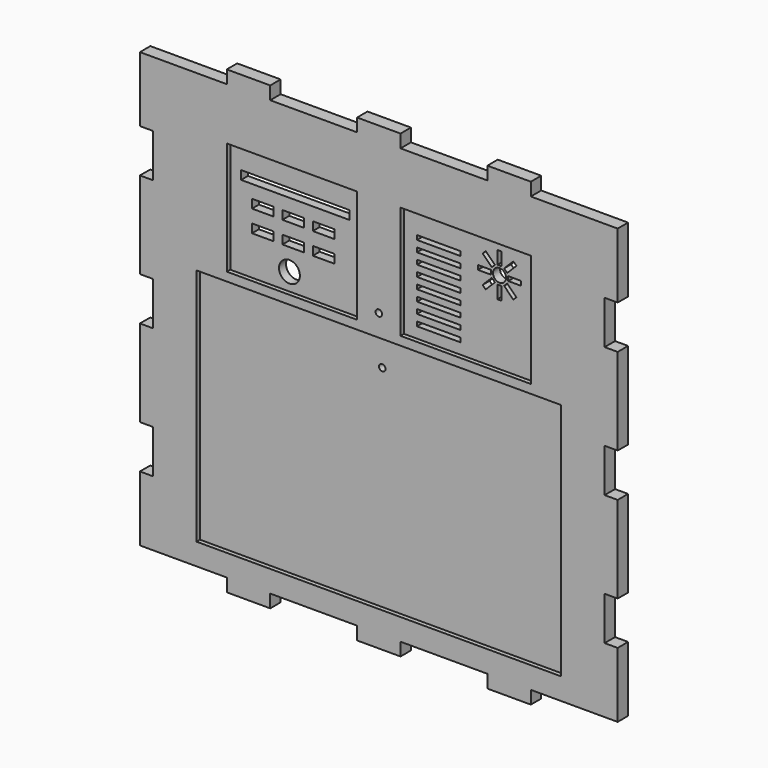
from build123d import *

# Parameters (mm, degrees)
F0_W     = 10
F0_H     = 3
F1_DEPTH = 3
F2_R     = 0.75
F2_W     = 5
F2_H     = 2
F2_R_2   = 2.4
F2_W_2   = 25
F2_W_3   = 10
F2_H_2   = 1
F2_R_3   = 1.5
F3_DEPTH = 3
F2_W_4   = 30
F2_H_3   = 26
F4_DEPTH = 1


# Not quite as in the source:
# - a feature names something its author has since deleted; it is built from what else it names


with BuildPart() as f1:
    # F0 (on Front) → F1 (new body)
    with BuildSketch(Plane.XZ):
        with Locations((-30, 51.5)):
            Rectangle(F0_W, F0_H)
        with Locations((0, 51.5)):
            Rectangle(F0_W, F0_H)
        with Locations((30, 51.5)):
            Rectangle(F0_W, F0_H)
        with Locations((-30, 48.5)):
            Rectangle(F0_W, F0_H)
        with Locations((0, 48.5)):
            Rectangle(F0_W, F0_H)
        with Locations((30, 48.5)):
            Rectangle(F0_W, F0_H)
        Polygon((-35, 50), (-55, 50), (-55, 35), (-52, 35), (-52, 25), (-55, 25), (-55, 5), (-52, 5), (-52, -5), (-55, -5), (-55, -25), (-52, -25), (-52, -35), (-55, -35), (-55, -50), (-35, -50), (-35, -47), (-25, -47), (-25, -50), (-5, -50), (-5, -47), (5, -47), (5, -50), (25, -50), (25, -47), (35, -47), (35, -50), (55, -50), (55, -35), (52, -35), (52, -25), (55, -25), (55, -5), (52, -5), (52, 5), (55, 5), (55, 25), (52, 25), (52, 35), (55, 35), (55, 50), (35, 50), (35, 47), (25, 47), (25, 50), (5, 50), (5, 47), (-5, 47), (-5, 50), (-25, 50), (-25, 47), (-35, 47), align=None)
        with Locations((30, -48.5)):
            Rectangle(F0_W, F0_H)
        with Locations((30, -51.5)):
            Rectangle(F0_W, F0_H)
        with Locations((0, -48.5)):
            Rectangle(F0_W, F0_H)
        with Locations((0, -51.5)):
            Rectangle(F0_W, F0_H)
        with Locations((-30, -48.5)):
            Rectangle(F0_W, F0_H)
        with Locations((-30, -51.5)):
            Rectangle(F0_W, F0_H)
    extrude(amount=F1_DEPTH)

    # F2 (on face) → F3 (cut)
    with BuildSketch(Plane.XZ.offset(3)):
        with Locations((0, 15)):
            Circle(F2_R)
        with Locations((-13.5, 22)):
            Rectangle(F2_W, F2_H)
        with Locations((-20.5, 22)):
            Rectangle(F2_W, F2_H)
        with Locations((-21.369388327, 16)):
            Circle(F2_R_2)
        with Locations((-27.5, 22)):
            Rectangle(F2_W, F2_H)
        with Locations((-27.5, 27)):
            Rectangle(F2_W, F2_H)
        with Locations((-20.5, 27)):
            Rectangle(F2_W, F2_H)
        with Locations((-13.5, 27)):
            Rectangle(F2_W, F2_H)
        with Locations((-20, 32)):
            Rectangle(F2_W_2, F2_H)
        with Locations((13, 32.5)):
            Rectangle(F2_W_3, F2_H_2)
        with Locations((13, 30)):
            Rectangle(F2_W_3, F2_H_2)
        with Locations((13, 27.5)):
            Rectangle(F2_W_3, F2_H_2)
        with Locations((13, 25)):
            Rectangle(F2_W_3, F2_H_2)
        with Locations((13, 22.5)):
            Rectangle(F2_W_3, F2_H_2)
        with Locations((13, 20)):
            Rectangle(F2_W_3, F2_H_2)
        with Locations((13, 17.5)):
            Rectangle(F2_W_3, F2_H_2)
        with Locations((13, 15)):
            Rectangle(F2_W_3, F2_H_2)
        with Locations((0, 3.5)):
            Circle(F2_R)
        Polygon((28.0606601718, 32.767766953), (28.4142135865, 32.4142135383), (28.767766953, 32.0606601718), (30.8890872965, 34.1819805153), (30.1819805153, 34.8890872965), align=None)
        Polygon((26.5, 33), (27, 33), (27.5, 33), (27.5, 36), (26.5, 36), align=None)
        Polygon((25.232233047, 32.0606601718), (25.5857864376, 32.4142135624), (25.9393398282, 32.767766953), (23.8180194847, 34.8890872965), (23.1109127035, 34.1819805153), align=None)
        Polygon((25, 30.5), (25, 31), (25, 31.5), (22, 31.5), (22, 30.5), align=None)
        Polygon((25.9393398282, 29.232233047), (25.5857864376, 29.5857864376), (25.232233047, 29.9393398282), (23.1109127035, 27.8180194847), (23.8180194847, 27.1109127035), align=None)
        Polygon((27.5, 29), (27, 29), (26.5, 29), (26.5, 26), (27.5, 26), align=None)
        Polygon((28.767766953, 29.9393398282), (28.4142135624, 29.5857864376), (28.0606601718, 29.232233047), (30.1819805153, 27.1109127035), (30.8890872965, 27.8180194847), align=None)
        Polygon((29, 31.5), (29, 31), (29, 30.5), (32, 30.5), (32, 31.5), align=None)
        with Locations((27, 31)):
            Circle(F2_R_3)
    extrude(amount=-F3_DEPTH, mode=Mode.SUBTRACT)

    # F2 (on face) → F4 (cut)
    with BuildSketch(Plane.XZ.offset(3)):
        with Locations((20, 25)):
            Rectangle(F2_W_4, F2_H_3)
        with Locations((13, 15)):
            Rectangle(F2_W_3, F2_H_2, mode=Mode.SUBTRACT)
        with Locations((13, 17.5)):
            Rectangle(F2_W_3, F2_H_2, mode=Mode.SUBTRACT)
        with Locations((13, 20)):
            Rectangle(F2_W_3, F2_H_2, mode=Mode.SUBTRACT)
        with Locations((13, 22.5)):
            Rectangle(F2_W_3, F2_H_2, mode=Mode.SUBTRACT)
        with Locations((13, 25)):
            Rectangle(F2_W_3, F2_H_2, mode=Mode.SUBTRACT)
        with Locations((13, 27.5)):
            Rectangle(F2_W_3, F2_H_2, mode=Mode.SUBTRACT)
        with Locations((13, 30)):
            Rectangle(F2_W_3, F2_H_2, mode=Mode.SUBTRACT)
        with Locations((13, 32.5)):
            Rectangle(F2_W_3, F2_H_2, mode=Mode.SUBTRACT)
        Polygon((26.5, 29), (27, 29), (27.5, 29), (27.5, 26), (26.5, 26), align=None, mode=Mode.SUBTRACT)
        Polygon((25.232233047, 29.9393398282), (25.5857864376, 29.5857864376), (25.9393398282, 29.232233047), (23.8180194847, 27.1109127035), (23.1109127035, 27.8180194847), align=None, mode=Mode.SUBTRACT)
        Polygon((25, 31.5), (25, 31), (25, 30.5), (22, 30.5), (22, 31.5), align=None, mode=Mode.SUBTRACT)
        with BuildLine():
            ThreePointArc((28.4142135865, 32.4142135383), (28.8477590715, 31.765366849), (29, 31))
            ThreePointArc((29, 31), (28.847759065, 30.2346331353), (28.4142135624, 29.5857864376))
            ThreePointArc((28.4142135624, 29.5857864376), (27.7653668647, 29.152240935), (27, 29))
            ThreePointArc((27, 29), (26.2346331353, 29.152240935), (25.5857864376, 29.5857864376))
            ThreePointArc((25.5857864376, 29.5857864376), (25.152240935, 30.2346331353), (25, 31))
            ThreePointArc((25, 31), (25.152240935, 31.7653668647), (25.5857864376, 32.4142135624))
            ThreePointArc((25.5857864376, 32.4142135624), (26.2346331353, 32.847759065), (27, 33))
            ThreePointArc((27, 33), (27.7653668805, 32.8477590585), (28.4142135865, 32.4142135383))
        make_face(mode=Mode.SUBTRACT)
        Polygon((25.9393398282, 32.767766953), (25.5857864376, 32.4142135624), (25.232233047, 32.0606601718), (23.1109127035, 34.1819805153), (23.8180194847, 34.8890872965), align=None, mode=Mode.SUBTRACT)
        Polygon((27.5, 33), (27, 33), (26.5, 33), (26.5, 36), (27.5, 36), align=None, mode=Mode.SUBTRACT)
        Polygon((28.0606601718, 29.232233047), (28.4142135624, 29.5857864376), (28.767766953, 29.9393398282), (30.8890872965, 27.8180194847), (30.1819805153, 27.1109127035), align=None, mode=Mode.SUBTRACT)
        Polygon((29, 30.5), (29, 31), (29, 31.5), (32, 31.5), (32, 30.5), align=None, mode=Mode.SUBTRACT)
        Polygon((28.767766953, 32.0606601718), (28.4142135865, 32.4142135383), (28.0606601718, 32.767766953), (30.1819805153, 34.8890872965), (30.8890872965, 34.1819805153), align=None, mode=Mode.SUBTRACT)
        with Locations((-20, 25)):
            Rectangle(F2_W_4, F2_H_3)
        with Locations((-21.369388327, 16)):
            Circle(F2_R_2, mode=Mode.SUBTRACT)
        with Locations((-27.5, 22)):
            Rectangle(F2_W, F2_H, mode=Mode.SUBTRACT)
        with Locations((-20.5, 22)):
            Rectangle(F2_W, F2_H, mode=Mode.SUBTRACT)
        with Locations((-13.5, 22)):
            Rectangle(F2_W, F2_H, mode=Mode.SUBTRACT)
        with Locations((-27.5, 27)):
            Rectangle(F2_W, F2_H, mode=Mode.SUBTRACT)
        with Locations((-20.5, 27)):
            Rectangle(F2_W, F2_H, mode=Mode.SUBTRACT)
        with Locations((-20, 32)):
            Rectangle(F2_W_2, F2_H, mode=Mode.SUBTRACT)
        with Locations((-13.5, 27)):
            Rectangle(F2_W, F2_H, mode=Mode.SUBTRACT)
        with BuildLine():
            ThreePointArc((28.4142135624, 29.5857864376), (28.847759065, 30.2346331353), (29, 31))
            ThreePointArc((29, 31), (28.8477590715, 31.765366849), (28.4142135865, 32.4142135383))
            ThreePointArc((28.4142135865, 32.4142135383), (27.7653668805, 32.8477590585), (27, 33))
            ThreePointArc((27, 33), (26.2346331353, 32.847759065), (25.5857864376, 32.4142135624))
            ThreePointArc((25.5857864376, 32.4142135624), (25.152240935, 31.7653668647), (25, 31))
            ThreePointArc((25, 31), (25.152240935, 30.2346331353), (25.5857864376, 29.5857864376))
            ThreePointArc((25.5857864376, 29.5857864376), (26.2346331353, 29.152240935), (27, 29))
            ThreePointArc((27, 29), (27.7653668647, 29.152240935), (28.4142135624, 29.5857864376))
        make_face()
        with Locations((27, 31)):
            Circle(F2_R_3, mode=Mode.SUBTRACT)
        Polygon((-35, 10), (-42, 10), (-42, -45), (42, -45), (42, 10), (35, 10), (5, 10), (-5, 10), align=None)
        with Locations((0, 3.5)):
            Circle(F2_R, mode=Mode.SUBTRACT)
    extrude(amount=-F4_DEPTH, mode=Mode.SUBTRACT)


solid = f1.part
